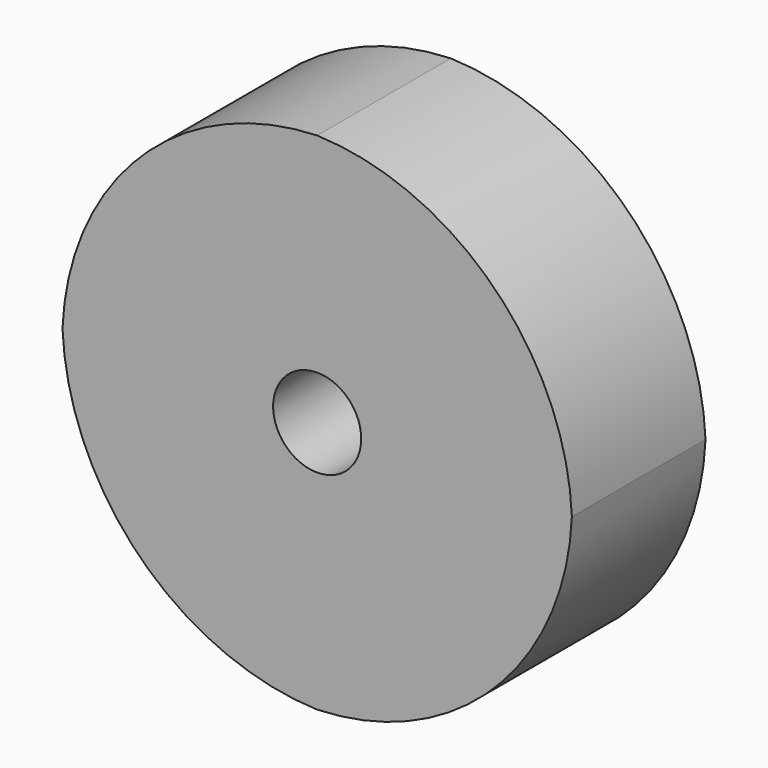
from build123d import *

# Parameters (mm, degrees)
F1_W        = 864.7019863129
F1_H        = 857.8115701675
F1_R        = 74.6623748118
F2_DEPTH    = 141.6553631425
F3_T1_DEPTH = 2521.5281199611


# Not quite as in the source:
# - a fillet or chamfer that OpenCascade refuses, or shapes differently, is made with other operations: its cross-section is extruded or revolved along the edge and cut away or added


with BuildPart() as f2:
    # F1 (on face) → F2 (new body, symmetric)
    with BuildSketch(Plane.XZ):
        Rectangle(F1_W, F1_H)
        Circle(F1_R, mode=Mode.SUBTRACT)
    extrude(amount=F2_DEPTH, both=True)

    # F3: fillet of radius 447.6434787352 on 4 edges, made by hand

    # F3_s2 → F3_t1 (cut)
    with BuildSketch(Plane.XZ.offset(-1260.7640599805)):
        with BuildLine():
            ThreePointArc((-15.2924855788, 428.9057850838), (301.2392537888, 297.7940457162), (432.3509931564, -18.7376936514))
            Line((432.3509931564, -18.7376936514), (432.3509931564, 428.9057850838))
            Line((432.3509931564, 428.9057850838), (-15.2924855788, 428.9057850838))
        make_face()
        with BuildLine():
            ThreePointArc((-15.2924855788, -428.9057850838), (301.2392537888, -297.7940457162), (432.3509931564, 18.7376936514))
            Line((432.3509931564, 18.7376936514), (432.3509931564, -428.9057850838))
            Line((432.3509931564, -428.9057850838), (-15.2924855788, -428.9057850838))
        make_face()
        with BuildLine():
            ThreePointArc((15.2924855788, -428.9057850838), (-301.2392537888, -297.7940457162), (-432.3509931564, 18.7376936514))
            Line((-432.3509931564, 18.7376936514), (-432.3509931564, -428.9057850838))
            Line((-432.3509931564, -428.9057850838), (15.2924855788, -428.9057850838))
        make_face()
        with BuildLine():
            ThreePointArc((-432.3509931564, -18.7376936514), (-301.2392537888, 297.7940457162), (15.2924855788, 428.9057850838))
            Line((15.2924855788, 428.9057850838), (-432.3509931564, 428.9057850838))
            Line((-432.3509931564, 428.9057850838), (-432.3509931564, -18.7376936514))
        make_face()
    extrude(amount=F3_T1_DEPTH, mode=Mode.SUBTRACT)


solid = f2.part
